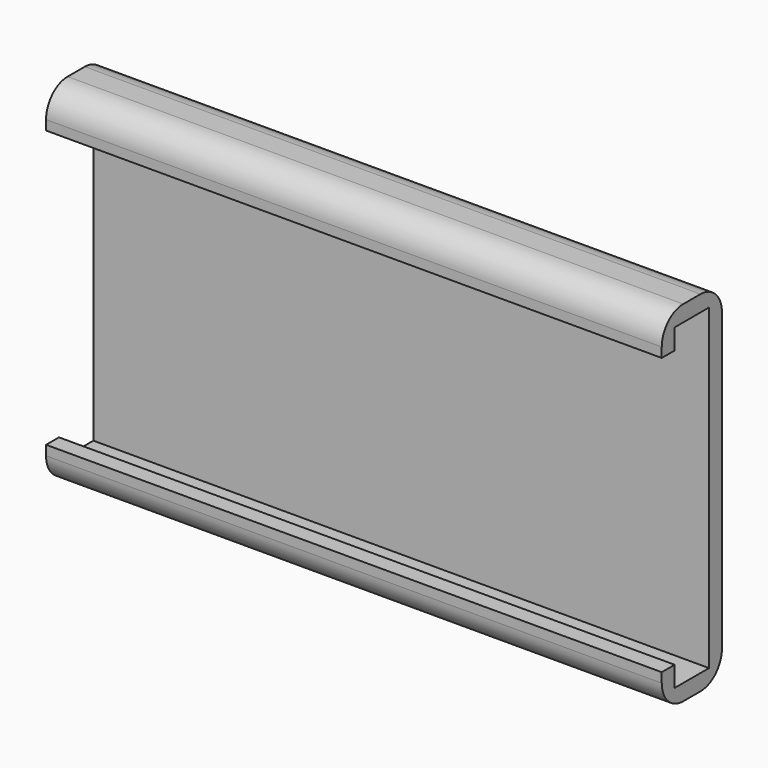
from build123d import *

# Parameters (mm, degrees)
F1_DEPTH      = 72.771
F1_DEPTH_BACK = 72.771
F2_R          = 0.9525
F3_DEPTH      = 2.794


# Not quite as in the source:
# - a length typed as a fraction of an inch, garbled in the dataset ("3 / 203.2 mm" for 3/8 in), is restored


with BuildPart() as f1:
    # F0 (on Right) → F1 (new body, two sides)
    with BuildSketch(Plane.YZ) as f1_sk:
        with BuildLine():
            Line((-8.008403407, 37.52215), (-8.008403407, 0))
            Line((-8.008403407, 0), (-8.008403407, -37.52215))
            Line((-8.008403407, -37.52215), (-18.168403407, -37.52215))
            Line((-18.168403407, -37.52215), (-18.168403407, -32.69615))
            Line((-18.168403407, -32.69615), (-21.978403407, -32.69615))
            Line((-21.978403407, -32.69615), (-21.978403407, -34.98215))
            ThreePointArc((-21.978403407, -34.98215), (-20.1185314675, -39.4722780605), (-15.628403407, -41.33215))
            Line((-15.628403407, -41.33215), (-10.548403407, -41.33215))
            ThreePointArc((-10.548403407, -41.33215), (-6.0582753465, -39.4722780605), (-4.198403407, -34.98215))
            Line((-4.198403407, -34.98215), (-4.198403407, 0))
            Line((-4.198403407, 0), (-4.198403407, 34.98215))
            ThreePointArc((-4.198403407, 34.98215), (-6.0582753465, 39.4722780605), (-10.548403407, 41.33215))
            Line((-10.548403407, 41.33215), (-15.628403407, 41.33215))
            ThreePointArc((-15.628403407, 41.33215), (-20.1185314675, 39.4722780605), (-21.978403407, 34.98215))
            Line((-21.978403407, 34.98215), (-21.978403407, 32.69615))
            Line((-21.978403407, 32.69615), (-18.168403407, 32.69615))
            Line((-18.168403407, 32.69615), (-18.168403407, 37.52215))
            Line((-18.168403407, 37.52215), (-8.008403407, 37.52215))
        make_face()
    extrude(amount=F1_DEPTH)
    extrude(f1_sk.sketch, amount=-F1_DEPTH_BACK)

    # F2 (on face) → F3 (cut)
    with BuildSketch(Plane(origin=(0, -4.198403407, 0), x_dir=(-1, 0, 0), z_dir=(0, 1, 0))):
        Circle(F2_R)
    extrude(amount=-F3_DEPTH, mode=Mode.SUBTRACT)


solid = f1.part
